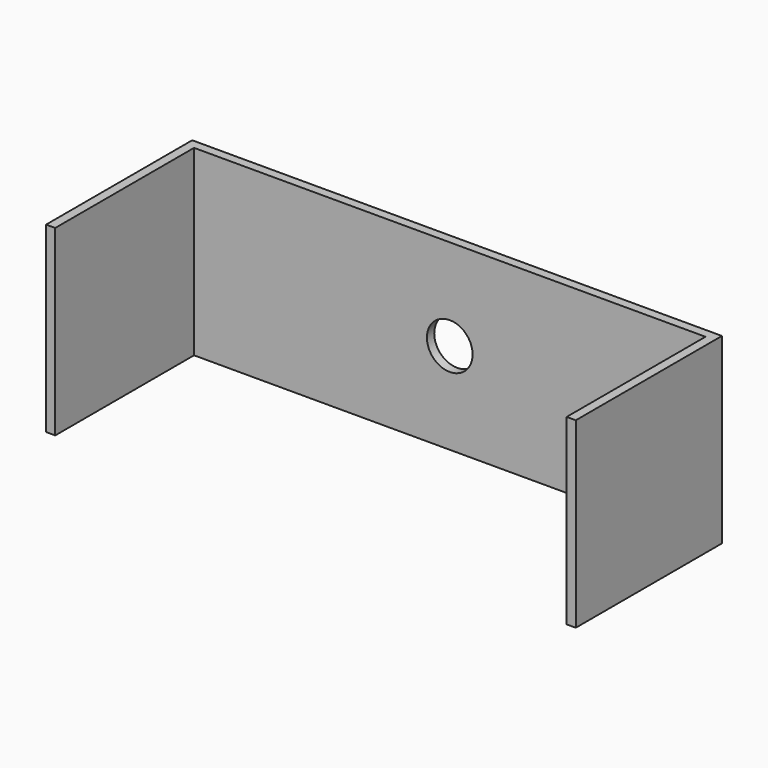
from build123d import *

# Parameters (mm, degrees)
F1_DEPTH = 12.7
F3_D     = 6.35
F3_DEPTH = 12.7
F3_TIP   = 1.9077324654


# Not quite as in the source:
# - a feature names something its author has since deleted; it is built from what else it names


with BuildPart() as f1:
    # F0 (on Top) → F1 (new body, symmetric)
    with BuildSketch(Plane.XY):
        Polygon((36.83, -12.7), (36.83, 12.7), (-36.83, 12.7), (-36.83, -12.7), (-35.56, -12.7), (-35.56, 11.43), (35.56, 11.43), (35.56, -12.7), align=None)
    extrude(amount=F1_DEPTH, both=True)

    # F3
    with Locations(Plane.XZ.offset(-11.43)):
        with Locations((0, 0)):
            Hole(F3_D / 2, depth=F3_DEPTH)
            with Locations((0, 0, -(F3_DEPTH + F3_TIP / 2))):  # 118° drill point
                Cone(0, F3_D / 2, F3_TIP, mode=Mode.SUBTRACT)


solid = f1.part
